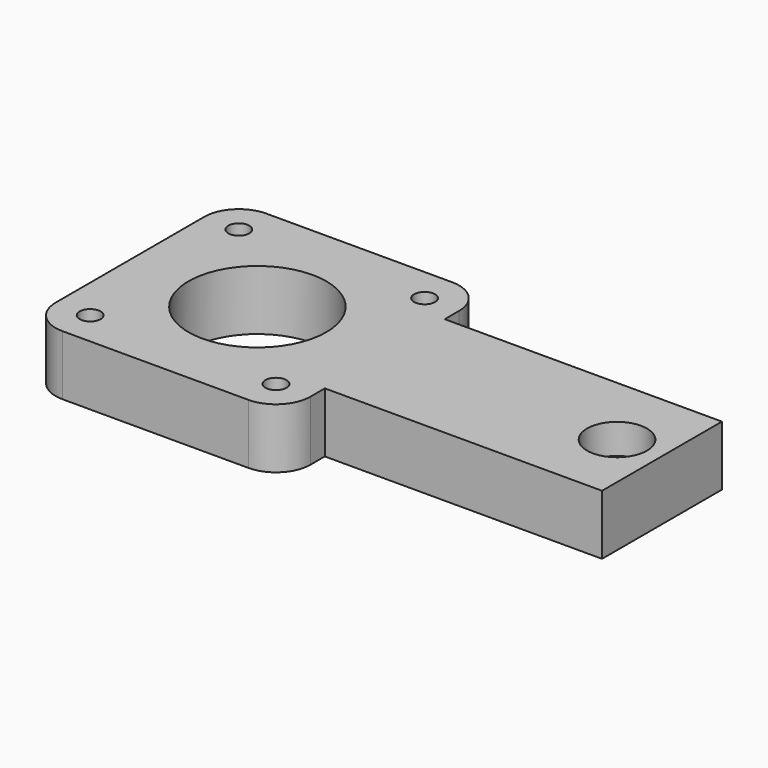
from build123d import *

# Parameters (mm, degrees)
F0_R     = 11.5
F0_R_2   = 1.75
F0_W     = 46.25
F0_H     = 25
F0_R_3   = 2.5
F1_DEPTH = 10
F2_R     = 5
F2_R_2   = 2.5
F3_DEPTH = 5


# Not quite as in the source:
# - a feature names something its author has since deleted; it is built from what else it names


with BuildPart() as f1:
    # F0 (on Top) → F1 (new body)
    with BuildSketch(Plane.XY):
        with BuildLine():
            Line((15.5000000202, 21.25), (-15.5, 21.25))
            ThreePointArc((-15.5, 21.25), (-11.4341360082, 19.5658639918), (-9.75, 15.5))
            ThreePointArc((-9.75, 15.5), (-15.5, 9.75), (-21.25, 15.5))
            Line((-21.25, 15.5), (-21.25, -15.4999999845))
            ThreePointArc((-21.25, -15.4999999845), (-15.4999999923, -9.75), (-9.75, -15.5))
            ThreePointArc((-9.75, -15.5), (-11.4341360082, -19.5658639918), (-15.5, -21.25))
            Line((-15.5, -21.25), (15.4999999923, -21.25))
            ThreePointArc((15.4999999923, -21.25), (11.4341360109, -11.4341360054), (21.25, -15.5))
            Line((21.25, -15.5), (21.25, -12.5))
            Line((21.25, -12.5), (21.25, 12.5))
            Line((21.25, 12.5), (21.25, 15.5))
            ThreePointArc((21.25, 15.5), (11.434136001, 11.4341360153), (15.5000000202, 21.25))
        make_face()
        Circle(F0_R, mode=Mode.SUBTRACT)
        with BuildLine():
            ThreePointArc((-9.75, -15.5), (-15.4999999923, -9.75), (-21.25, -15.4999999845))
            ThreePointArc((-21.25, -15.4999999845), (-19.5658639973, -19.5658639864), (-15.5, -21.25))
            ThreePointArc((-15.5, -21.25), (-11.4341360082, -19.5658639918), (-9.75, -15.5))
        make_face()
        with Locations((-15.5, -15.5)):
            Circle(F0_R_2, mode=Mode.SUBTRACT)
        with BuildLine():
            ThreePointArc((-9.75, 15.5), (-11.4341360082, 19.5658639918), (-15.5, 21.25))
            ThreePointArc((-15.5, 21.25), (-19.5658639918, 19.5658639918), (-21.25, 15.5))
            ThreePointArc((-21.25, 15.5), (-15.5, 9.75), (-9.75, 15.5))
        make_face()
        with Locations((-15.5, 15.5)):
            Circle(F0_R_2, mode=Mode.SUBTRACT)
        with BuildLine():
            ThreePointArc((21.25, 15.5), (19.565863999, 19.5658639847), (15.5000000202, 21.25))
            ThreePointArc((15.5000000202, 21.25), (11.434136001, 11.4341360153), (21.25, 15.5))
        make_face()
        with Locations((15.5, 15.5)):
            Circle(F0_R_2, mode=Mode.SUBTRACT)
        with BuildLine():
            ThreePointArc((21.25, -15.5), (11.4341360109, -11.4341360054), (15.4999999923, -21.25))
            ThreePointArc((15.4999999923, -21.25), (19.5658639891, -19.5658639946), (21.25, -15.5))
        make_face()
        with Locations((15.5, -15.5)):
            Circle(F0_R_2, mode=Mode.SUBTRACT)
        with Locations((44.375, 0)):
            Rectangle(F0_W, F0_H)
        with Locations((60, 0)):
            Circle(F0_R_3, mode=Mode.SUBTRACT)
    extrude(amount=F1_DEPTH)

    # F2 (on face) → F3 (cut)
    with BuildSketch(Plane.XY.offset(10)):
        with Locations((60, 0)):
            Circle(F2_R)
        with Locations((60, 0)):
            Circle(F2_R_2, mode=Mode.SUBTRACT)
    extrude(amount=-F3_DEPTH, mode=Mode.SUBTRACT)


solid = f1.part
